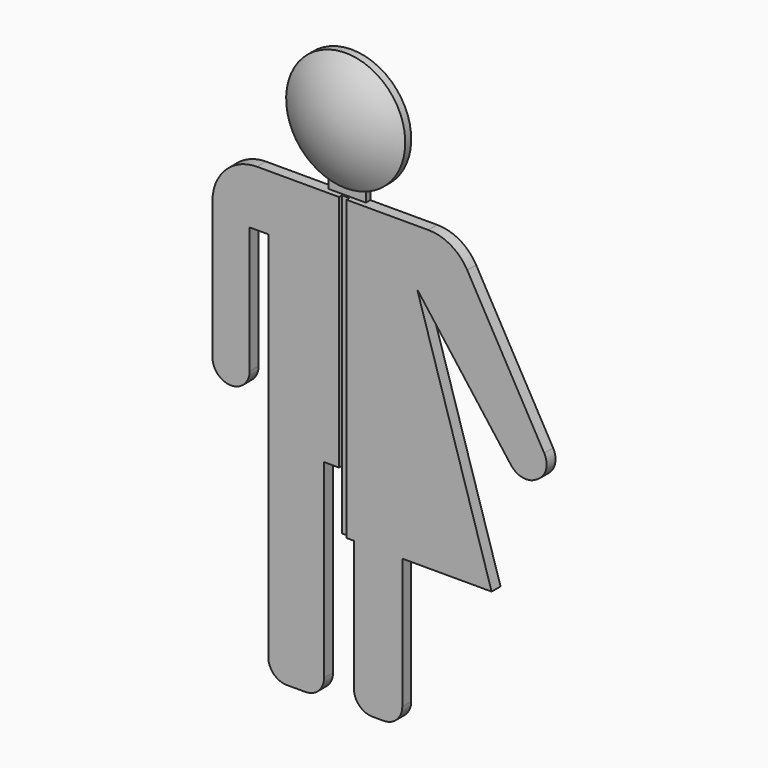
from build123d import *

# Parameters (mm, degrees)
F0_W     = 10
F0_H     = 6
F0_W_2   = 13
F0_H_2   = 16
F0_W_3   = 4
F0_H_3   = 40
F1_DEPTH = 3
F2_R     = 4.99999
F3_DEPTH = 1.5
F4_R     = 12
F8_DEPTH = 1


# Not quite as in the source:
# - a fillet or chamfer is up to 0.001 mm smaller than in the source, because OpenCascade refuses the exact size


with BuildPart() as f1:
    # F0 (on Front) → F1 (new body)
    with BuildSketch(Plane.XZ):
        with Locations((0, 44)):
            Rectangle(F0_W, F0_H)
        Polygon((-5, 41), (-5, 47), (-20, 47), (-20, 32), (-20, -7), (-20, -73), (-5, -73), (-5, -17), (-1, -17), (3, -17), (16, -17), (16, -33), (20, -33), (20, 32), (20, 47), (5, 47), (5, 41), align=None)
        Polygon((-20, 32), (-20, 47), (-35, 47), (-35, -7), (-25, -7), (-25, 32), align=None)
        Polygon((40, -33), (20, 32), (20, -33), align=None)
        Polygon((30, 47), (20, 47), (20, 32), (47.8857678969, -4.9239762223), (56.5894716006, 0), align=None)
        with Locations((9.5, -25)):
            Rectangle(F0_W_2, F0_H_2)
        with Locations((1, -25)):
            Rectangle(F0_W_3, F0_H_2)
        with Locations((9.5, -53)):
            Rectangle(F0_W_2, F0_H_3)
    extrude(amount=F1_DEPTH)

    # F2 (radius 5 in the source; OpenCascade refuses exactly that, so slightly less here)
    f2_edges = [f1.edges().sort_by_distance(p)[0] for p in [
        (56.589472, -1.5, 0),
        (47.885768, -1.5, -4.923976),
        (-25, -1.5, -7),
        (-35, -1.5, -7),
        (16, -1.5, -73),
        (3, -1.5, -73),
        (-20, -1.5, -73),
        (-5, -1.5, -73),
    ]]
    fillet(f2_edges, radius=F2_R)

    # F4
    f4_edges = [f1.edges().sort_by_distance(p)[0] for p in [
        (30, -1.5, 47),
        (-35, -1.5, 47),
    ]]
    fillet(f4_edges, radius=F4_R)

    # F7 (on face) → F8 (cut)
    with BuildSketch(Plane.XZ.offset(3)):
        Polygon((-1, -17), (-1, -33), (1, -33), (1, 47), (-1, 47), align=None)
    extrude(amount=-F8_DEPTH, mode=Mode.SUBTRACT)


with BuildPart() as f3:
    # F0 (on Front) → F3 (new body)
    with BuildSketch(Plane.XZ):
        with BuildLine():
            ThreePointArc((5, 50.8578643763), (0, 50), (-5, 50.8578643763))
            Line((-5, 50.8578643763), (-5, 47))
            Line((-5, 47), (5, 47))
            Line((5, 47), (5, 50.8578643763))
        make_face()
    extrude(amount=F3_DEPTH)

    # F5 (on Right) → F6 (revolve)
    with BuildSketch(Plane.YZ):
        with BuildLine():
            Line((0, 49), (0, 65))
            Line((0, 65), (-7, 65))
            ThreePointArc((-7, 65), (-5.7208873828, 56.6184726929), (-2, 49))
            Line((-2, 49), (0, 49))
        make_face()
    revolve(axis=Axis((0, -3.5, 65), (0, -1, 0)))


solid = Compound([f1.part, f3.part])
